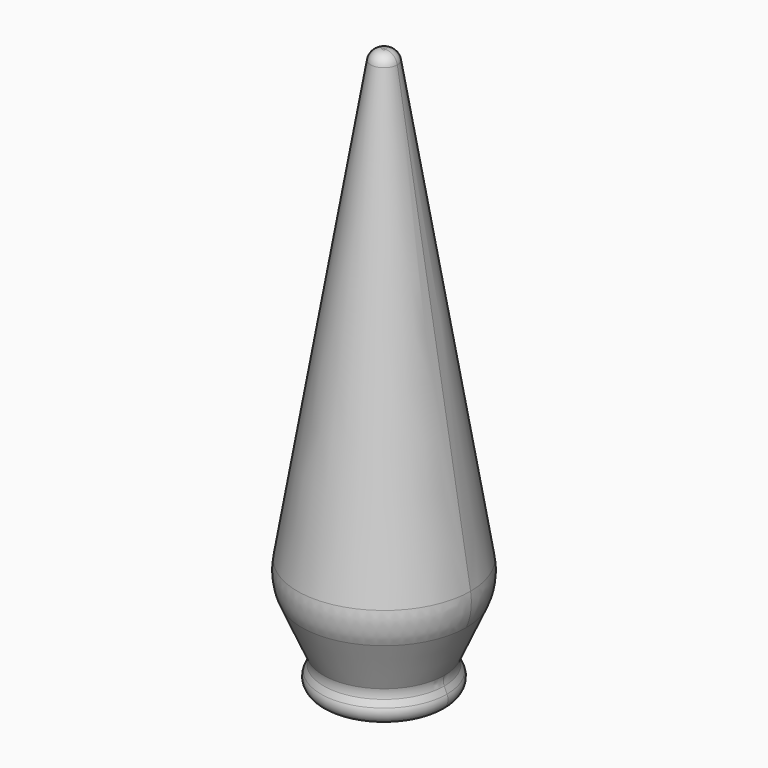
from build123d import *
from build123d import SkipClean  # not in build123d's __all__

# Parameters (mm, degrees)
F1_ANGLE = 180
F3_R     = 3
F4_R     = 3
F5_R     = 15


with BuildPart() as f1:
    # F0 (on Front) → F1 (revolve)
    with BuildSketch(Plane.XZ):
        Polygon((15, -18), (23, 0), (3, 120), (0, 120), (0, -25), (18, -25), align=None)
    revolve(axis=Axis((0, 0, 130.329349637), (0, 0, 1)), revolution_arc=F1_ANGLE)

    # F2: F1 across plane


with BuildPart() as f1_1:
    add(f1.part, clean=False)
    with SkipClean():  # cleaning this boolean's faces spoils the solid; the shape is the same uncleaned
        add(f1.part.mirror(Plane.XZ), clean=False)

    # F3
    f3_edges = [f1_1.edges().sort_by_distance(p)[0] for p in [
        (0, 3, 120),
        (0, -3, 120),
    ]]
    fillet(f3_edges, radius=F3_R)

    # F4
    f4_edges = [f1_1.edges().sort_by_distance(p)[0] for p in [
        (0, 15, -18),
        (0, -15, -18),
        (0, 18, -25),
        (0, -18, -25),
    ]]
    fillet(f4_edges, radius=F4_R)

    # F5
    f5_edges = [f1_1.edges().sort_by_distance(p)[0] for p in [
        (0, 23, 0),
        (0, -23, 0),
    ]]
    fillet(f5_edges, radius=F5_R)


solid = f1_1.part
